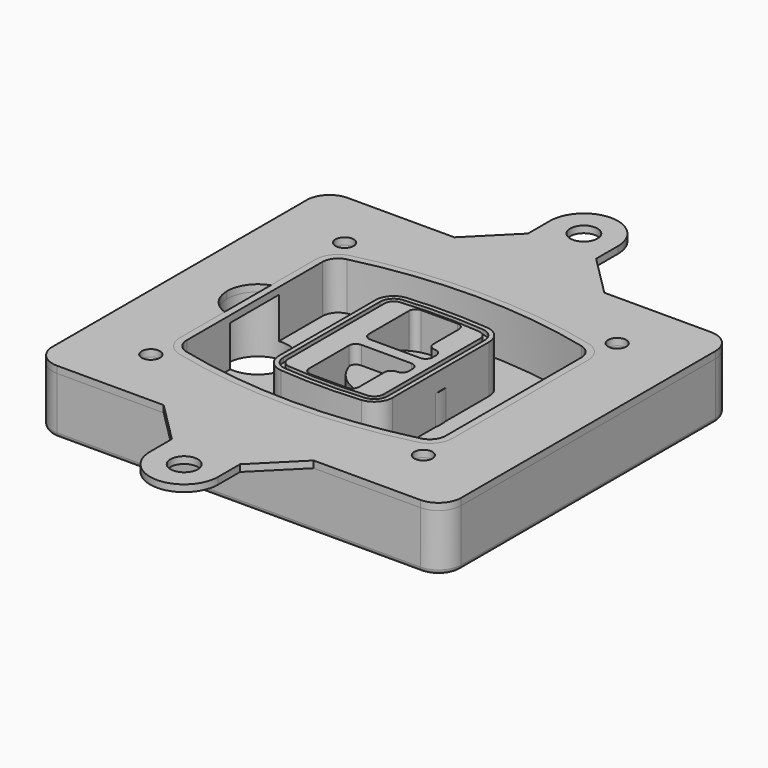
from build123d import *

# Parameters (mm, degrees)
F0_R      = 4
F1_DEPTH  = 25
F2_DEPTH  = 3
F3_DEPTH  = 18
F5_DEPTH  = 21
F6_DEPTH  = 2
F8_DEPTH  = 20
F9_DEPTH  = 16
F10_DEPTH = 25
F7_R      = 6
F7_R_2    = 4
F11_DEPTH = 6
F13_DEPTH = 9
F15_R     = 2
F16_R     = 4
F16_R_2   = 6
F17_DEPTH = 3


# Not quite as in the source:
# - a feature of the source that left no trace in its solid (it failed there, or was rolled back) is left out
# - a feature names something its author has since deleted; it is built from what else it names


with BuildPart() as f1:
    # F0 (on Top) → F1 (new body)
    with BuildSketch(Plane.XY):
        with BuildLine():
            ThreePointArc((-90, -70), (-87.0710678119, -77.0710678119), (-80, -80))
            Line((-80, -80), (80, -80))
            ThreePointArc((80, -80), (87.0710678119, -77.0710678119), (90, -70))
            Line((90, -70), (90, 70))
            ThreePointArc((90, 70), (87.0710678119, 77.0710678119), (80, 80))
            Line((80, 80), (-80, 80))
            ThreePointArc((-80, 80), (-87.0710678119, 77.0710678119), (-90, 70))
            Line((-90, 70), (-90, -70))
        make_face()
        with Locations((-60, -53.3333333333)):
            Circle(F0_R, mode=Mode.SUBTRACT)
        with Locations((60, -53.3333333333)):
            Circle(F0_R, mode=Mode.SUBTRACT)
        with Locations((-60, 53.3333333333)):
            Circle(F0_R, mode=Mode.SUBTRACT)
        with BuildLine():
            ThreePointArc((-64, 37.2990447398), (-61.0143011354, 45.9411029726), (-53.3306899286, 50.8970778549))
            ThreePointArc((-53.3306899286, 50.8970778549), (0, 57.3333333333), (53.3306899286, 50.8970778549))
            ThreePointArc((53.3306899286, 50.8970778549), (61.0143011354, 45.9411029726), (64, 37.2990447398))
            Line((64, 37.2990447398), (64, -37.2990447398))
            ThreePointArc((64, -37.2990447398), (61.0143011354, -45.9411029726), (53.3306899286, -50.8970778549))
            ThreePointArc((53.3306899286, -50.8970778549), (0, -57.3333333333), (-53.3306899286, -50.8970778549))
            ThreePointArc((-53.3306899286, -50.8970778549), (-61.0143011354, -45.9411029726), (-64, -37.2990447398))
            Line((-64, -37.2990447398), (-64, 37.2990447398))
        make_face(mode=Mode.SUBTRACT)
        with Locations((60, 53.3333333333)):
            Circle(F0_R, mode=Mode.SUBTRACT)
        with BuildLine():
            ThreePointArc((53.3306899286, 50.8970778549), (0, 57.3333333333), (-53.3306899286, 50.8970778549))
            ThreePointArc((-53.3306899286, 50.8970778549), (-61.0143011354, 45.9411029726), (-64, 37.2990447398))
            Line((-64, 37.2990447398), (-64, -37.2990447398))
            ThreePointArc((-64, -37.2990447398), (-61.0143011354, -45.9411029726), (-53.3306899286, -50.8970778549))
            ThreePointArc((-53.3306899286, -50.8970778549), (0, -57.3333333333), (53.3306899286, -50.8970778549))
            ThreePointArc((53.3306899286, -50.8970778549), (61.0143011354, -45.9411029726), (64, -37.2990447398))
            Line((64, -37.2990447398), (64, 37.2990447398))
            ThreePointArc((64, 37.2990447398), (61.0143011354, 45.9411029726), (53.3306899286, 50.8970778549))
        make_face()
        with BuildLine():
            Line((-60, -37.2990447398), (-60, 37.2990447398))
            ThreePointArc((-60, 37.2990447398), (-57.8673579538, 43.4719434775), (-52.3790642347, 47.0119255363))
            ThreePointArc((-52.3790642347, 47.0119255363), (0, 53.3333333333), (52.3790642347, 47.0119255363))
            ThreePointArc((52.3790642347, 47.0119255363), (57.8673579538, 43.4719434775), (60, 37.2990447398))
            Line((60, 37.2990447398), (60, -37.2990447398))
            ThreePointArc((60, -37.2990447398), (57.8673579538, -43.4719434775), (52.3790642347, -47.0119255363))
            ThreePointArc((52.3790642347, -47.0119255363), (0, -53.3333333333), (-52.3790642347, -47.0119255363))
            ThreePointArc((-52.3790642347, -47.0119255363), (-57.8673579538, -43.4719434775), (-60, -37.2990447398))
        make_face(mode=Mode.SUBTRACT)
        with BuildLine():
            ThreePointArc((-52.3790642347, 47.0119255363), (-57.8673579538, 43.4719434775), (-60, 37.2990447398))
            Line((-60, 37.2990447398), (-60, -37.2990447398))
            ThreePointArc((-60, -37.2990447398), (-57.8673579538, -43.4719434775), (-52.3790642347, -47.0119255363))
            ThreePointArc((-52.3790642347, -47.0119255363), (0, -53.3333333333), (52.3790642347, -47.0119255363))
            ThreePointArc((52.3790642347, -47.0119255363), (57.8673579538, -43.4719434775), (60, -37.2990447398))
            Line((60, -37.2990447398), (60, 37.2990447398))
            ThreePointArc((60, 37.2990447398), (57.8673579538, 43.4719434775), (52.3790642347, 47.0119255363))
            ThreePointArc((52.3790642347, 47.0119255363), (0, 53.3333333333), (-52.3790642347, 47.0119255363))
        make_face()
        with BuildLine():
            ThreePointArc((51.6653449643, 44.0980612973), (55.5071505677, 41.6200738562), (57, 37.2990447398))
            Line((57, 37.2990447398), (57, -37.2990447398))
            ThreePointArc((57, -37.2990447398), (55.5071505677, -41.6200738562), (51.6653449643, -44.0980612973))
            ThreePointArc((51.6653449643, -44.0980612973), (0, -50.3333333333), (-51.6653449643, -44.0980612973))
            ThreePointArc((-51.6653449643, -44.0980612973), (-55.5071505677, -41.6200738562), (-57, -37.2990447398))
            Line((-57, -37.2990447398), (-57, 37.2990447398))
            ThreePointArc((-57, 37.2990447398), (-55.5071505677, 41.6200738562), (-51.6653449643, 44.0980612973))
            ThreePointArc((-51.6653449643, 44.0980612973), (0, 50.3333333333), (51.6653449643, 44.0980612973))
        make_face(mode=Mode.SUBTRACT)
        with BuildLine():
            Line((57, -37.2990447398), (57, 37.2990447398))
            ThreePointArc((57, 37.2990447398), (55.5071505677, 41.6200738562), (51.6653449643, 44.0980612973))
            ThreePointArc((51.6653449643, 44.0980612973), (0, 50.3333333333), (-51.6653449643, 44.0980612973))
            ThreePointArc((-51.6653449643, 44.0980612973), (-55.5071505677, 41.6200738562), (-57, 37.2990447398))
            Line((-57, 37.2990447398), (-57, -37.2990447398))
            ThreePointArc((-57, -37.2990447398), (-55.5071505677, -41.6200738562), (-51.6653449643, -44.0980612973))
            ThreePointArc((-51.6653449643, -44.0980612973), (0, -50.3333333333), (51.6653449643, -44.0980612973))
            ThreePointArc((51.6653449643, -44.0980612973), (55.5071505677, -41.6200738562), (57, -37.2990447398))
        make_face()
    extrude(amount=-F1_DEPTH)

    # F0 (on Top) → F2 (join)
    with BuildSketch(Plane.XY):
        with BuildLine():
            ThreePointArc((-52.3790642347, 47.0119255363), (-57.8673579538, 43.4719434775), (-60, 37.2990447398))
            Line((-60, 37.2990447398), (-60, -37.2990447398))
            ThreePointArc((-60, -37.2990447398), (-57.8673579538, -43.4719434775), (-52.3790642347, -47.0119255363))
            ThreePointArc((-52.3790642347, -47.0119255363), (0, -53.3333333333), (52.3790642347, -47.0119255363))
            ThreePointArc((52.3790642347, -47.0119255363), (57.8673579538, -43.4719434775), (60, -37.2990447398))
            Line((60, -37.2990447398), (60, 37.2990447398))
            ThreePointArc((60, 37.2990447398), (57.8673579538, 43.4719434775), (52.3790642347, 47.0119255363))
            ThreePointArc((52.3790642347, 47.0119255363), (0, 53.3333333333), (-52.3790642347, 47.0119255363))
        make_face()
        with BuildLine():
            ThreePointArc((51.6653449643, 44.0980612973), (55.5071505677, 41.6200738562), (57, 37.2990447398))
            Line((57, 37.2990447398), (57, -37.2990447398))
            ThreePointArc((57, -37.2990447398), (55.5071505677, -41.6200738562), (51.6653449643, -44.0980612973))
            ThreePointArc((51.6653449643, -44.0980612973), (0, -50.3333333333), (-51.6653449643, -44.0980612973))
            ThreePointArc((-51.6653449643, -44.0980612973), (-55.5071505677, -41.6200738562), (-57, -37.2990447398))
            Line((-57, -37.2990447398), (-57, 37.2990447398))
            ThreePointArc((-57, 37.2990447398), (-55.5071505677, 41.6200738562), (-51.6653449643, 44.0980612973))
            ThreePointArc((-51.6653449643, 44.0980612973), (0, 50.3333333333), (51.6653449643, 44.0980612973))
        make_face(mode=Mode.SUBTRACT)
    extrude(amount=F2_DEPTH)

    # F0 (on Top) → F3 (cut)
    with BuildSketch(Plane.XY):
        with BuildLine():
            Line((57, -37.2990447398), (57, 37.2990447398))
            ThreePointArc((57, 37.2990447398), (55.5071505677, 41.6200738562), (51.6653449643, 44.0980612973))
            ThreePointArc((51.6653449643, 44.0980612973), (0, 50.3333333333), (-51.6653449643, 44.0980612973))
            ThreePointArc((-51.6653449643, 44.0980612973), (-55.5071505677, 41.6200738562), (-57, 37.2990447398))
            Line((-57, 37.2990447398), (-57, -37.2990447398))
            ThreePointArc((-57, -37.2990447398), (-55.5071505677, -41.6200738562), (-51.6653449643, -44.0980612973))
            ThreePointArc((-51.6653449643, -44.0980612973), (0, -50.3333333333), (51.6653449643, -44.0980612973))
            ThreePointArc((51.6653449643, -44.0980612973), (55.5071505677, -41.6200738562), (57, -37.2990447398))
        make_face()
    extrude(amount=-F3_DEPTH, mode=Mode.SUBTRACT)

    # F4 (on face) → F5 (join, through all)
    with BuildSketch(Plane.XY.offset(3)):
        with BuildLine():
            ThreePointArc((-25, -26.587695628), (-22.8992979869, -31.9912392117), (-17.7004291845, -34.5569740744))
            ThreePointArc((-17.7004291845, -34.5569740744), (0, -35.3333333333), (17.7004291845, -34.5569740744))
            ThreePointArc((17.7004291845, -34.5569740744), (22.8992979869, -31.9912392117), (25, -26.587695628))
            Line((25, -26.587695628), (25, 26.587695628))
            ThreePointArc((25, 26.587695628), (22.8992979869, 31.9912392117), (17.7004291845, 34.5569740744))
            ThreePointArc((17.7004291845, 34.5569740744), (0, 35.3333333333), (-17.7004291845, 34.5569740744))
            ThreePointArc((-17.7004291845, 34.5569740744), (-22.8992979869, 31.9912392117), (-25, 26.587695628))
            Line((-25, 26.587695628), (-25, -26.587695628))
        make_face()
        with BuildLine():
            ThreePointArc((17.5253218884, 32.5646544628), (21.4244734902, 30.6403533158), (23, 26.587695628))
            Line((23, 26.587695628), (23, -26.587695628))
            ThreePointArc((23, -26.587695628), (21.4244734902, -30.6403533158), (17.5253218884, -32.5646544628))
            ThreePointArc((17.5253218884, -32.5646544628), (0, -33.3333333333), (-17.5253218884, -32.5646544628))
            ThreePointArc((-17.5253218884, -32.5646544628), (-21.4244734902, -30.6403533158), (-23, -26.587695628))
            Line((-23, -26.587695628), (-23, 26.587695628))
            ThreePointArc((-23, 26.587695628), (-21.4244734902, 30.6403533158), (-17.5253218884, 32.5646544628))
            ThreePointArc((-17.5253218884, 32.5646544628), (0, 33.3333333333), (17.5253218884, 32.5646544628))
        make_face(mode=Mode.SUBTRACT)
        with BuildLine():
            Line((23, -26.587695628), (23, 26.587695628))
            ThreePointArc((23, 26.587695628), (21.4244734902, 30.6403533158), (17.5253218884, 32.5646544628))
            ThreePointArc((17.5253218884, 32.5646544628), (0, 33.3333333333), (-17.5253218884, 32.5646544628))
            ThreePointArc((-17.5253218884, 32.5646544628), (-21.4244734902, 30.6403533158), (-23, 26.587695628))
            Line((-23, 26.587695628), (-23, -26.587695628))
            ThreePointArc((-23, -26.587695628), (-21.4244734902, -30.6403533158), (-17.5253218884, -32.5646544628))
            ThreePointArc((-17.5253218884, -32.5646544628), (0, -33.3333333333), (17.5253218884, -32.5646544628))
            ThreePointArc((17.5253218884, -32.5646544628), (21.4244734902, -30.6403533158), (23, -26.587695628))
        make_face()
        with BuildLine():
            ThreePointArc((17.3502145923, 30.5723348512), (19.9496489934, 29.2894674198), (21, 26.587695628))
            Line((21, 26.587695628), (21, -26.587695628))
            ThreePointArc((21, -26.587695628), (19.9496489934, -29.2894674198), (17.3502145923, -30.5723348512))
            ThreePointArc((17.3502145923, -30.5723348512), (0, -31.3333333333), (-17.3502145923, -30.5723348512))
            ThreePointArc((-17.3502145923, -30.5723348512), (-19.9496489934, -29.2894674198), (-21, -26.587695628))
            Line((-21, -26.587695628), (-21, 26.587695628))
            ThreePointArc((-21, 26.587695628), (-19.9496489934, 29.2894674198), (-17.3502145923, 30.5723348512))
            ThreePointArc((-17.3502145923, 30.5723348512), (0, 31.3333333333), (17.3502145923, 30.5723348512))
        make_face(mode=Mode.SUBTRACT)
        with BuildLine():
            Line((21, -26.587695628), (21, 26.587695628))
            ThreePointArc((21, 26.587695628), (19.9496489934, 29.2894674198), (17.3502145923, 30.5723348512))
            ThreePointArc((17.3502145923, 30.5723348512), (0, 31.3333333333), (-17.3502145923, 30.5723348512))
            ThreePointArc((-17.3502145923, 30.5723348512), (-19.9496489934, 29.2894674198), (-21, 26.587695628))
            Line((-21, 26.587695628), (-21, -26.587695628))
            ThreePointArc((-21, -26.587695628), (-19.9496489934, -29.2894674198), (-17.3502145923, -30.5723348512))
            ThreePointArc((-17.3502145923, -30.5723348512), (0, -31.3333333333), (17.3502145923, -30.5723348512))
            ThreePointArc((17.3502145923, -30.5723348512), (19.9496489934, -29.2894674198), (21, -26.587695628))
        make_face()
        with BuildLine():
            Line((-8, -2.5), (14, -2.5))
            ThreePointArc((14, -2.5), (16.1213203436, -3.3786796564), (17, -5.5))
            Line((17, -5.5), (17, -7.5))
            ThreePointArc((17, -7.5), (16.1213203436, -9.6213203436), (14, -10.5))
            ThreePointArc((14, -10.5), (11.8786796564, -11.3786796564), (11, -13.5))
            Line((11, -13.5), (11, -27.5))
            ThreePointArc((11, -27.5), (10.1213203436, -29.6213203436), (8, -30.5))
            Line((8, -30.5), (-8, -30.5))
            ThreePointArc((-8, -30.5), (-10.1213203436, -29.6213203436), (-11, -27.5))
            Line((-11, -27.5), (-11, -5.5))
            ThreePointArc((-11, -5.5), (-10.1213203436, -3.3786796564), (-8, -2.5))
        make_face(mode=Mode.SUBTRACT)
        with BuildLine():
            ThreePointArc((-8, 2.5), (-10.1213203436, 3.3786796564), (-11, 5.5))
            Line((-11, 5.5), (-11, 27.5))
            ThreePointArc((-11, 27.5), (-10.1213203436, 29.6213203436), (-8, 30.5))
            Line((-8, 30.5), (8, 30.5))
            ThreePointArc((8, 30.5), (10.1213203436, 29.6213203436), (11, 27.5))
            Line((11, 27.5), (11, 13.5))
            ThreePointArc((11, 13.5), (11.8786796564, 11.3786796564), (14, 10.5))
            ThreePointArc((14, 10.5), (16.1213203436, 9.6213203436), (17, 7.5))
            Line((17, 7.5), (17, 5.5))
            ThreePointArc((17, 5.5), (16.1213203436, 3.3786796564), (14, 2.5))
            Line((14, 2.5), (-8, 2.5))
        make_face(mode=Mode.SUBTRACT)
    extrude(amount=-F5_DEPTH)

    # F4 (on face) → F6 (cut)
    with BuildSketch(Plane.XY.offset(3)):
        with BuildLine():
            Line((23, -26.587695628), (23, 26.587695628))
            ThreePointArc((23, 26.587695628), (21.4244734902, 30.6403533158), (17.5253218884, 32.5646544628))
            ThreePointArc((17.5253218884, 32.5646544628), (0, 33.3333333333), (-17.5253218884, 32.5646544628))
            ThreePointArc((-17.5253218884, 32.5646544628), (-21.4244734902, 30.6403533158), (-23, 26.587695628))
            Line((-23, 26.587695628), (-23, -26.587695628))
            ThreePointArc((-23, -26.587695628), (-21.4244734902, -30.6403533158), (-17.5253218884, -32.5646544628))
            ThreePointArc((-17.5253218884, -32.5646544628), (0, -33.3333333333), (17.5253218884, -32.5646544628))
            ThreePointArc((17.5253218884, -32.5646544628), (21.4244734902, -30.6403533158), (23, -26.587695628))
        make_face()
        with BuildLine():
            ThreePointArc((17.3502145923, 30.5723348512), (19.9496489934, 29.2894674198), (21, 26.587695628))
            Line((21, 26.587695628), (21, -26.587695628))
            ThreePointArc((21, -26.587695628), (19.9496489934, -29.2894674198), (17.3502145923, -30.5723348512))
            ThreePointArc((17.3502145923, -30.5723348512), (0, -31.3333333333), (-17.3502145923, -30.5723348512))
            ThreePointArc((-17.3502145923, -30.5723348512), (-19.9496489934, -29.2894674198), (-21, -26.587695628))
            Line((-21, -26.587695628), (-21, 26.587695628))
            ThreePointArc((-21, 26.587695628), (-19.9496489934, 29.2894674198), (-17.3502145923, 30.5723348512))
            ThreePointArc((-17.3502145923, 30.5723348512), (0, 31.3333333333), (17.3502145923, 30.5723348512))
        make_face(mode=Mode.SUBTRACT)
    extrude(amount=-F6_DEPTH, mode=Mode.SUBTRACT)

    # F7 (on face) → F8 (join)
    with BuildSketch(Plane(origin=(0, 0, -25), x_dir=(1, 0, 0), z_dir=(0, 0, -1))):
        with BuildLine():
            ThreePointArc((-6.71157564, 0), (6.7567035675, 13.4682792075), (20.224982775, 0))
            Line((20.224982775, 0), (25.224982775, 0))
            ThreePointArc((25.224982775, 0), (6.7567035675, 18.4682792075), (-11.71157564, 0))
            Line((-11.71157564, 0), (-6.71157564, 0))
        make_face()
        with BuildLine():
            Line((-6.71157564, 0), (20.224982775, 0))
            ThreePointArc((20.224982775, 0), (6.7567035675, 13.4682792075), (-6.71157564, 0))
        make_face()
        with BuildLine():
            ThreePointArc((-6.71157564, 0), (6.7567035675, -13.4682792075), (20.224982775, 0))
            Line((20.224982775, 0), (-6.71157564, 0))
        make_face()
        with BuildLine():
            Line((25.224982775, 0), (20.224982775, 0))
            ThreePointArc((20.224982775, 0), (6.7567035675, -13.4682792075), (-6.71157564, 0))
            Line((-6.71157564, 0), (-11.71157564, 0))
            ThreePointArc((-11.71157564, 0), (6.7567035675, -18.4682792075), (25.224982775, 0))
        make_face()
    extrude(amount=-F8_DEPTH)

    # F7 (on face) → F9 (cut)
    with BuildSketch(Plane(origin=(0, 0, -25), x_dir=(1, 0, 0), z_dir=(0, 0, -1))):
        with BuildLine():
            Line((-6.71157564, 0), (20.224982775, 0))
            ThreePointArc((20.224982775, 0), (6.7567035675, 13.4682792075), (-6.71157564, 0))
        make_face()
        with BuildLine():
            ThreePointArc((-6.71157564, 0), (6.7567035675, -13.4682792075), (20.224982775, 0))
            Line((20.224982775, 0), (-6.71157564, 0))
        make_face()
    extrude(amount=-F9_DEPTH, mode=Mode.SUBTRACT)

    # F7 (on face) → F10 (cut)
    with BuildSketch(Plane(origin=(0, 0, -25), x_dir=(1, 0, 0), z_dir=(0, 0, -1))):
        with BuildLine():
            Line((-69.0318229325, 0), (-42.0952645175, 0))
            ThreePointArc((-42.0952645175, 0), (-55.563543725, 13.4682792075), (-69.0318229325, 0))
        make_face()
        with BuildLine():
            ThreePointArc((-69.0318229325, 0), (-55.563543725, -13.4682792075), (-42.0952645175, 0))
            Line((-42.0952645175, 0), (-69.0318229325, 0))
        make_face()
    extrude(amount=-F10_DEPTH, mode=Mode.SUBTRACT)

    # F7 (on face) → F11 (cut)
    with BuildSketch(Plane(origin=(0, 0, -25), x_dir=(1, 0, 0), z_dir=(0, 0, -1))):
        with Locations((60, -53.3333333333)):
            Circle(F7_R)
        with Locations((60, -53.3333333333)):
            Circle(F7_R_2, mode=Mode.SUBTRACT)
        with Locations((-60, -53.3333333333)):
            Circle(F7_R)
        with Locations((-60, -53.3333333333)):
            Circle(F7_R_2, mode=Mode.SUBTRACT)
        with Locations((-60, 53.3333333333)):
            Circle(F7_R)
        with Locations((-60, 53.3333333333)):
            Circle(F7_R_2, mode=Mode.SUBTRACT)
        with Locations((60, 53.3333333333)):
            Circle(F7_R)
        with Locations((60, 53.3333333333)):
            Circle(F7_R_2, mode=Mode.SUBTRACT)
    extrude(amount=-F11_DEPTH, mode=Mode.SUBTRACT)

    # F12 (on face) → F13 (cut, through all)
    with BuildSketch(Plane(origin=(0, 0, -9), x_dir=(1, 0, 0), z_dir=(0, 0, -1))):
        with BuildLine():
            ThreePointArc((20.224982775, 0), (20.1663399806, 1.2554664788), (19.9909222755, 2.5))
            Line((19.9909222755, 2.5), (14, 2.5))
            ThreePointArc((14, 2.5), (16.1213203436, 3.3786796564), (17, 5.5))
            Line((17, 5.5), (17, 7.5))
            ThreePointArc((17, 7.5), (16.1213203436, 9.6213203436), (14, 10.5))
            ThreePointArc((14, 10.5), (12.1627255951, 11.1284134507), (11.0951631559, 12.750384826))
            ThreePointArc((11.0951631559, 12.750384826), (11.0476113807, 12.7664660322), (11, 12.7823698976))
            Line((11, 12.7823698976), (11, -12.7823698976))
            ThreePointArc((11, -12.7823698976), (11.0476113807, -12.7664660322), (11.0951631559, -12.750384826))
            ThreePointArc((11.0951631559, -12.750384826), (12.1627255951, -11.1284134507), (14, -10.5))
            ThreePointArc((14, -10.5), (16.1213203436, -9.6213203436), (17, -7.5))
            Line((17, -7.5), (17, -5.5))
            ThreePointArc((17, -5.5), (16.1213203436, -3.3786796564), (14, -2.5))
            Line((14, -2.5), (19.9909222755, -2.5))
            ThreePointArc((19.9909222755, -2.5), (20.1663399806, -1.2554664788), (20.224982775, 0))
        make_face()
    extrude(amount=F13_DEPTH, mode=Mode.SUBTRACT)

    # F15
    f15_edges = [f1.edges().sort_by_distance(p)[0] for p in [
        (0, -80, -25),
        (-87.071068, -77.071068, -25),
        (-90, 0, -25),
        (-87.071068, 77.071068, -25),
        (87.071068, -77.071068, -25),
        (0, 80, -25),
        (90, 0, -25),
        (87.071068, 77.071068, -25),
    ]]
    fillet(f15_edges, radius=F15_R)


with BuildPart() as f17:
    # F16 (on face) → F17 (new body, through all)
    with BuildSketch(Plane.XY):
        with BuildLine():
            Line((33, 80), (-33, 80))
            Line((-33, 80), (-80, 80))
            ThreePointArc((-80, 80), (-87.0710678119, 77.0710678119), (-90, 70))
            Line((-90, 70), (-90, -70))
            ThreePointArc((-90, -70), (-87.0710678119, -77.0710678119), (-80, -80))
            Line((-80, -80), (-33, -80))
            Line((-33, -80), (33, -80))
            Line((33, -80), (80, -80))
            ThreePointArc((80, -80), (87.0710678119, -77.0710678119), (90, -70))
            Line((90, -70), (90, 70))
            ThreePointArc((90, 70), (87.0710678119, 77.0710678119), (80, 80))
            Line((80, 80), (33, 80))
        make_face()
        with Locations((-60, -53.3333333333)):
            Circle(F16_R, mode=Mode.SUBTRACT)
        with BuildLine():
            Line((-60, 12.7166190685), (-60, 37.2990447398))
            ThreePointArc((-60, 37.2990447398), (-57.8673579538, 43.4719434775), (-52.3790642347, 47.0119255363))
            ThreePointArc((-52.3790642347, 47.0119255363), (0, 53.3333333333), (52.3790642347, 47.0119255363))
            ThreePointArc((52.3790642347, 47.0119255363), (57.8673579538, 43.4719434775), (60, 37.2990447398))
            Line((60, 37.2990447398), (60, -37.2990447398))
            ThreePointArc((60, -37.2990447398), (57.8673579538, -43.4719434775), (52.3790642347, -47.0119255363))
            ThreePointArc((52.3790642347, -47.0119255363), (0, -53.3333333333), (-52.3790642347, -47.0119255363))
            ThreePointArc((-52.3790642347, -47.0119255363), (-57.8673579538, -43.4719434775), (-60, -37.2990447398))
            Line((-60, -37.2990447398), (-60, -12.7166190685))
            ThreePointArc((-60, -12.7166190685), (-66.5441169481, -7.798817635), (-69.0318229325, 0))
            ThreePointArc((-69.0318229325, 0), (-66.5441169481, 7.798817635), (-60, 12.7166190685))
        make_face(mode=Mode.SUBTRACT)
        with Locations((60, -53.3333333333)):
            Circle(F16_R, mode=Mode.SUBTRACT)
        with Locations((-60, 53.3333333333)):
            Circle(F16_R, mode=Mode.SUBTRACT)
        with Locations((60, 53.3333333333)):
            Circle(F16_R, mode=Mode.SUBTRACT)
        with BuildLine():
            Line((33, -80), (-33, -80))
            Line((-33, -80), (-15, -98))
            Line((-15, -98), (-15, -110))
            ThreePointArc((-15, -110), (0, -125), (15, -110))
            Line((15, -110), (15, -98))
            Line((15, -98), (33, -80))
        make_face()
        with Locations((0, -110)):
            Circle(F16_R_2, mode=Mode.SUBTRACT)
        with BuildLine():
            Line((-15, 98), (-33, 80))
            Line((-33, 80), (33, 80))
            Line((33, 80), (15, 98))
            Line((15, 98), (15, 110))
            ThreePointArc((15, 110), (0, 125), (-15, 110))
            Line((-15, 110), (-15, 98))
        make_face()
        with Locations((0, 110)):
            Circle(F16_R_2, mode=Mode.SUBTRACT)
    extrude(amount=F17_DEPTH)


solid = Compound([f1.part, f17.part])
